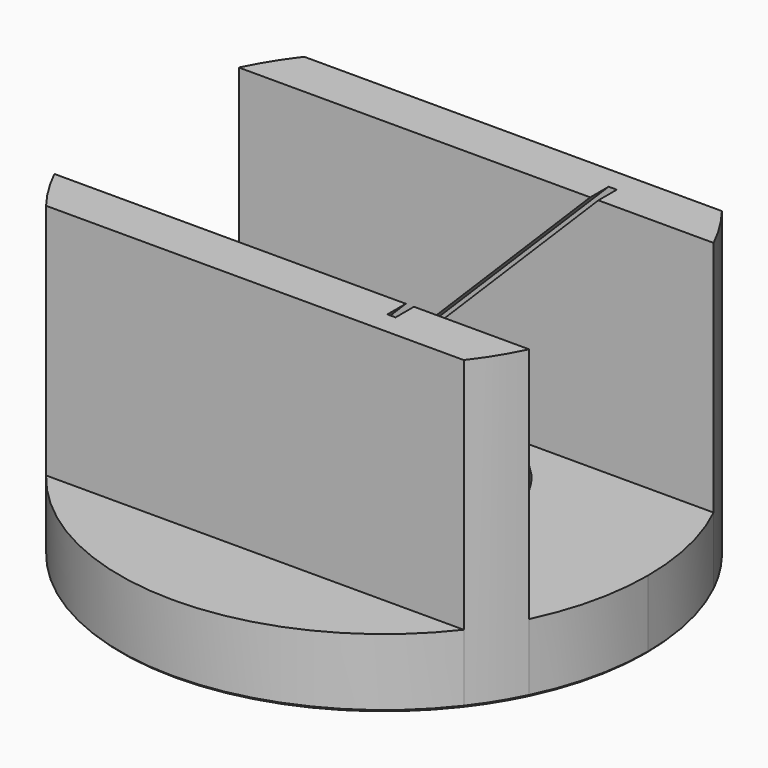
from build123d import *
from build123d import SkipClean  # not in build123d's __all__

# Parameters (mm, degrees)
F1_DEPTH = 6
F2_DEPTH = 26.6
F5_DEPTH = 0.5
F7_SIZE  = 0.2


# Not quite as in the source:
# - a feature names something its author has since deleted; it is built from what else it names


with BuildPart() as f1:
    # F0 (on Top) → F1 (new body)
    with BuildSketch(Plane.XY):
        with BuildLine():
            ThreePointArc((20.6012135565, -10), (22.3179052606, -5.1304098061), (22.9, 0))
            ThreePointArc((22.9, 0), (22.3179052606, 5.1304098061), (20.6012135565, 10))
            Line((20.6012135565, 10), (-3.73e-08, 10))
            ThreePointArc((-3.73e-08, 10), (7.0710677987, 7.0710678251), (10, 0))
            ThreePointArc((10, 0), (7.0710678119, -7.0710678119), (0, -10))
            Line((0, -10), (20.6012135565, -10))
        make_face()
        with BuildLine():
            Line((-3.73e-08, 10), (20.6012135565, 10))
            ThreePointArc((20.6012135565, 10), (19.464672656, 12.063851723), (18.1220859726, 14))
            Line((18.1220859726, 14), (-18.1220859726, 14))
            ThreePointArc((-18.1220859726, 14), (-19.464672656, 12.063851723), (-20.6012135565, 10))
            Line((-20.6012135565, 10), (-16, 10))
            Line((-16, 10), (-3.73e-08, 10))
        make_face()
        with BuildLine():
            ThreePointArc((18.1220859726, -14), (19.464672656, -12.063851723), (20.6012135565, -10))
            Line((20.6012135565, -10), (0, -10))
            Line((0, -10), (-16, -10))
            Line((-16, -10), (-20.6012135565, -10))
            ThreePointArc((-20.6012135565, -10), (-19.464672656, -12.063851723), (-18.1220859726, -14))
            Line((-18.1220859726, -14), (18.1220859726, -14))
        make_face()
        with BuildLine():
            Line((-18.1220859726, 14), (18.1220859726, 14))
            ThreePointArc((18.1220859726, 14), (0, 22.9), (-18.1220859726, 14))
        make_face()
        with BuildLine():
            ThreePointArc((-18.1220859726, -14), (0, -22.9), (18.1220859726, -14))
            Line((18.1220859726, -14), (-18.1220859726, -14))
        make_face()
        with BuildLine():
            Line((-16, -10), (-16, 10))
            Line((-16, 10), (-20.6012135565, 10))
            ThreePointArc((-20.6012135565, 10), (-22.9, 0), (-20.6012135565, -10))
            Line((-20.6012135565, -10), (-16, -10))
        make_face()
        with BuildLine():
            ThreePointArc((0, -10), (-10, -1.87e-08), (-3.73e-08, 10))
            Line((-3.73e-08, 10), (-16, 10))
            Line((-16, 10), (-16, -10))
            Line((-16, -10), (0, -10))
        make_face()
    extrude(amount=F1_DEPTH)

    # F0 (on Top) → F2 (join)
    with BuildSketch(Plane.XY):
        with BuildLine():
            Line((-3.73e-08, 10), (20.6012135565, 10))
            ThreePointArc((20.6012135565, 10), (19.464672656, 12.063851723), (18.1220859726, 14))
            Line((18.1220859726, 14), (-18.1220859726, 14))
            ThreePointArc((-18.1220859726, 14), (-19.464672656, 12.063851723), (-20.6012135565, 10))
            Line((-20.6012135565, 10), (-16, 10))
            Line((-16, 10), (-3.73e-08, 10))
        make_face()
        with BuildLine():
            ThreePointArc((18.1220859726, -14), (19.464672656, -12.063851723), (20.6012135565, -10))
            Line((20.6012135565, -10), (0, -10))
            Line((0, -10), (-16, -10))
            Line((-16, -10), (-20.6012135565, -10))
            ThreePointArc((-20.6012135565, -10), (-19.464672656, -12.063851723), (-18.1220859726, -14))
            Line((-18.1220859726, -14), (18.1220859726, -14))
        make_face()
    with SkipClean():  # cleaning this boolean's faces spoils the solid; the shape is the same uncleaned
        extrude(amount=F2_DEPTH)


with BuildPart() as f5:
    # F4 (on line) → F5 (new body)
    with BuildSketch(Plane(origin=(-8, 0, 8), x_dir=(0.7071067812, 0, 0.7071067812), z_dir=(0.7071067812, 0, -0.7071067812))):
        Polygon((-2.8284271247, -12), (-2.8284271247, -10), (-2.8284271247, 10), (-2.8284271247, 12), (-3.8284271247, 12), (-3.8284271247, -12), align=None)
        Polygon((-2.8284271247, 10), (-2.8284271247, -10), (-2.8284271247, -12), (26.3043722601, -12), (26.3043722601, -10), (26.3043722601, 10), (26.3043722601, 12), (-2.8284271247, 12), align=None)
        Polygon((26.3043722601, -10), (26.3043722601, -12), (28.3043722601, -12), (28.3043722601, 12), (26.3043722601, 12), (26.3043722601, 10), align=None)
    extrude(amount=-F5_DEPTH)


with BuildPart() as f1_1:
    add(f1.part, clean=False)

    # F6: cut F5
    add(f5.part, mode=Mode.SUBTRACT)

    # F7
    f7_edges = [f1_1.edges().sort_by_distance(p)[0] for p in [
        (-22.9, 0, 0),
    ]]
    chamfer(f7_edges, length=F7_SIZE)


solid = f1_1.part
